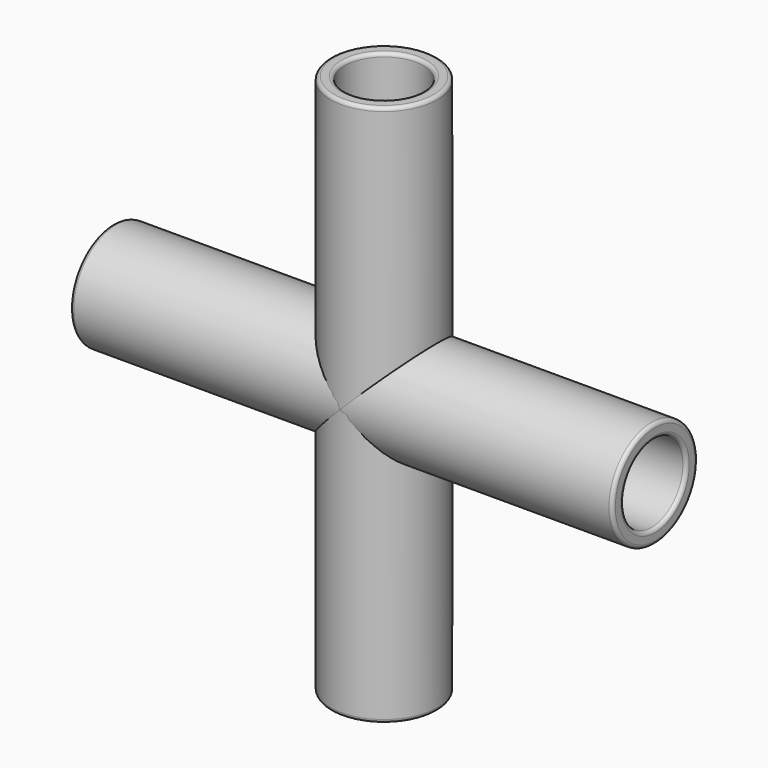
from build123d import *

# Parameters (mm, degrees)
F0_R     = 15
F0_R_2   = 11
F1_DEPTH = 76.2
F3_COUNT = 2
F3_ANGLE = 90
F5_R     = 1
F5_2_R   = 1
F4_R     = 10.9957996476
F6_DEPTH = 146.05
F7_R     = 11.0029340594
F8_DEPTH = 104.14


with BuildPart() as f1:
    # F0 (on Top) → F1 (new body, symmetric)
    with BuildSketch(Plane.XY):
        Circle(F0_R)
        Circle(F0_R_2, mode=Mode.SUBTRACT)
    extrude(amount=F1_DEPTH, both=True)


with BuildPart() as f3_1:
    # F3: instance of F1
    add(f1.part.rotate(Axis((0, -3.5612788051, 0), (0, -1, 0)), 1 * F3_ANGLE / (F3_COUNT - 1)))

    # F5#2
    f5_2_edges = [f3_1.edges().sort_by_distance(p)[0] for p in [
        (-76.2, 0, -11),
        (-76.2, 0, -15),
        (76.2, 0, -11),
        (76.2, 0, -15),
    ]]
    fillet(f5_2_edges, radius=F5_2_R)

    # F7 (on face) → F8 (cut)
    with BuildSketch(Plane(origin=(0, 0, -76.2), x_dir=(1, 0, 0), z_dir=(0, 0, -1))):
        Circle(F7_R)
    extrude(amount=-F8_DEPTH, mode=Mode.SUBTRACT)


with BuildPart() as f1_1:
    add(f1.part)

    # F5
    f5_edges = [f1_1.edges().sort_by_distance(p)[0] for p in [
        (-11, 0, 76.2),
        (-15, 0, 76.2),
        (-15, 0, -76.2),
        (-11, 0, -76.2),
    ]]
    fillet(f5_edges, radius=F5_R)

    # F4 (on face) → F6 (cut)
    with BuildSketch(Plane.YZ.offset(76.2)):
        Circle(F4_R)
    extrude(amount=-F6_DEPTH, mode=Mode.SUBTRACT)


solid = Compound([f3_1.part, f1_1.part])
